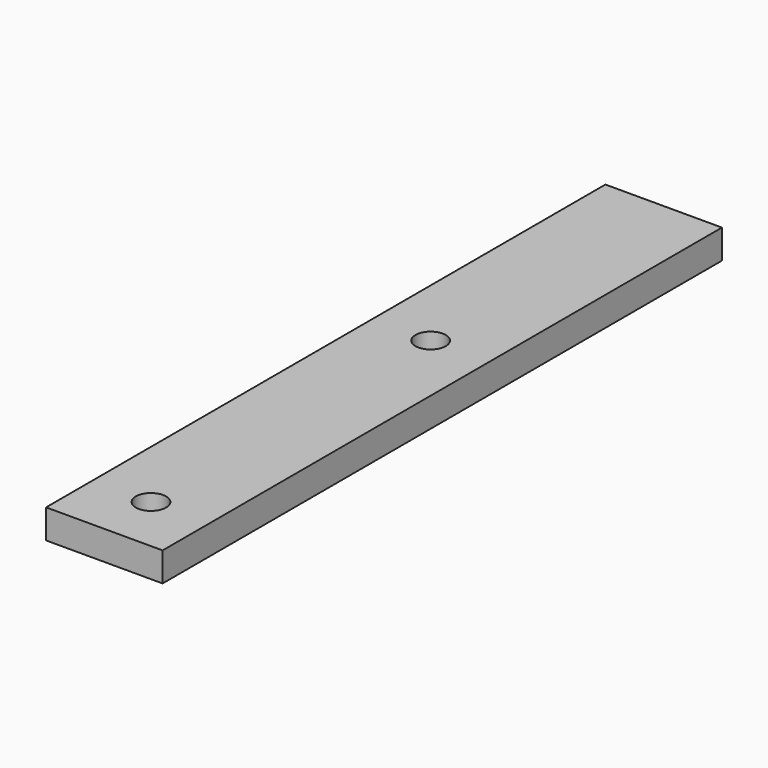
from build123d import *

# Parameters (mm, degrees)
F0_W     = 12.7
F0_H     = 76.2
F0_R     = 1.651
F1_DEPTH = 3.175


# Not quite as in the source:
# - a length typed as a fraction of an inch, garbled in the dataset ("3 / 203.2 mm" for 3/8 in), is restored


with BuildPart() as f1:
    # F0 (on Top) → F1 (new body)
    with BuildSketch(Plane.XY):
        with Locations((6.35, 38.1)):
            Rectangle(F0_W, F0_H)
        with Locations((6.35, 6.35)):
            Circle(F0_R, mode=Mode.SUBTRACT)
        with Locations((6.35, 44.45)):
            Circle(F0_R, mode=Mode.SUBTRACT)
    extrude(amount=F1_DEPTH)


solid = f1.part
